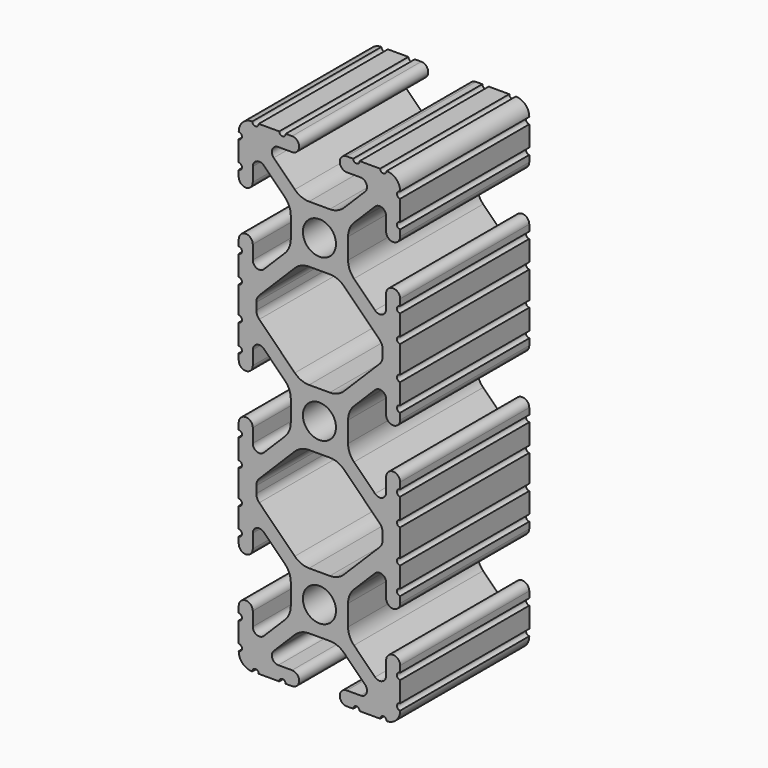
from build123d import *

# Parameters (mm, degrees)
F1_DEPTH = 25.4


# Not quite as in the source:
# - ends of sketch curves that miss each other by under 0.0002 mm in the source are joined


with BuildPart() as f1:
    # F0 (on Front) → F1 (new body)
    with BuildSketch(Plane.XZ):
        with BuildLine():
            ThreePointArc((-9.5504, 38.1), (-10.0584, 37.592), (-10.5664, 38.1))
            ThreePointArc((-10.5664, 38.1), (-12.0826749161, 37.4826749161), (-12.699997541, 35.9664000298))
            ThreePointArc((-12.699997541, 35.9664000298), (-12.192, 35.4584), (-12.7, 34.9504))
            Line((-12.7, 34.9504), (-12.7, 31.7246))
            ThreePointArc((-12.7, 31.7246), (-12.192, 31.2166), (-12.7, 30.7086))
            Line((-12.7, 30.7086), (-12.7, 29.7023028))
            ThreePointArc((-12.7, 29.7023028), (-11.5951, 28.5974028), (-10.4902, 29.7023028))
            Line((-10.4902, 29.7023028), (-10.4902, 31.8747902))
            ThreePointArc((-10.4902, 31.8747902), (-9.8630063673, 32.813451805), (-8.7557795103, 32.5932106897))
            Line((-8.7557795103, 32.5932106897), (-5.4384448, 29.2758622))
            ThreePointArc((-5.4384448, 29.2758622), (-4.7501824843, 28.2458268978), (-4.5085, 27.030807))
            Line((-4.5085, 27.030807), (-4.5085, 23.769193))
            ThreePointArc((-4.5085, 23.769193), (-4.7501824843, 22.5541731022), (-5.4384359697, 21.5241289697))
            Line((-5.4384359697, 21.5241289697), (-8.7557864, 18.2067962))
            ThreePointArc((-8.7557864, 18.2067962), (-9.8630063673, 17.986548195), (-10.4902, 18.9252098))
            Line((-10.4902, 18.9252098), (-10.4902, 21.0976972))
            ThreePointArc((-10.4902, 21.0976972), (-11.5951, 22.2025972), (-12.7, 21.0976972))
            Line((-12.7, 21.0976972), (-12.7, 20.0914))
            ThreePointArc((-12.7, 20.0914), (-12.192, 19.5834), (-12.7, 19.0754))
            Line((-12.7, 19.0754), (-12.7, 15.8496))
            ThreePointArc((-12.7, 15.8496), (-12.192, 15.3416), (-12.7, 14.8336))
            Line((-12.7, 14.8336), (-12.7, 10.5664))
            ThreePointArc((-12.7, 10.5664), (-12.192, 10.0584), (-12.7, 9.5504))
            Line((-12.7, 9.5504), (-12.7, 6.3246))
            ThreePointArc((-12.7, 6.3246), (-12.192, 5.8166), (-12.7, 5.3086))
            Line((-12.7, 5.3086), (-12.7, 4.3023028))
            ThreePointArc((-12.7, 4.3023028), (-11.5951, 3.1974028), (-10.4902, 4.3023028))
            Line((-10.4902, 4.3023028), (-10.4902, 6.4747902))
            ThreePointArc((-10.4902, 6.4747902), (-9.8630063673, 7.413451805), (-8.7557795103, 7.1932106897))
            Line((-8.7557795103, 7.1932106897), (-5.4384448, 3.8758622))
            ThreePointArc((-5.4384448, 3.8758622), (-4.7501824843, 2.8458268978), (-4.5085, 1.630807))
            Line((-4.5085, 1.630807), (-4.5085, -1.630807))
            ThreePointArc((-4.5085, -1.630807), (-4.7501824843, -2.8458268978), (-5.4384359697, -3.8758710303))
            Line((-5.4384359697, -3.8758710303), (-8.7557864, -7.1932038))
            ThreePointArc((-8.7557864, -7.1932038), (-9.8630063673, -7.413451805), (-10.4902, -6.4747902))
            Line((-10.4902, -6.4747902), (-10.4902, -4.3023028))
            ThreePointArc((-10.4902, -4.3023028), (-11.5951, -3.1974028), (-12.7, -4.3023028))
            Line((-12.7, -4.3023028), (-12.7, -5.3086))
            ThreePointArc((-12.7, -5.3086), (-12.192, -5.8166), (-12.7, -6.3246))
            Line((-12.7, -6.3246), (-12.7, -9.5504))
            ThreePointArc((-12.7, -9.5504), (-12.192, -10.0584), (-12.7, -10.5664))
            Line((-12.7, -10.5664), (-12.7, -14.8336))
            ThreePointArc((-12.7, -14.8336), (-12.192, -15.3416), (-12.7, -15.8496))
            Line((-12.7, -15.8496), (-12.7, -19.0754))
            ThreePointArc((-12.7, -19.0754), (-12.192, -19.5834), (-12.7, -20.0914))
            Line((-12.7, -20.0914), (-12.7, -21.0976972))
            ThreePointArc((-12.7, -21.0976972), (-11.5951, -22.2025972), (-10.4902, -21.0976972))
            Line((-10.4902, -21.0976972), (-10.4902, -18.9252098))
            ThreePointArc((-10.4902, -18.9252098), (-9.8630063673, -17.986548195), (-8.7557795103, -18.2067893103))
            Line((-8.7557795103, -18.2067893103), (-5.4384448, -21.5241378))
            ThreePointArc((-5.4384448, -21.5241378), (-4.7501824843, -22.5541731022), (-4.5085, -23.769193))
            Line((-4.5085, -23.769193), (-4.5085, -27.030807))
            ThreePointArc((-4.5085, -27.030807), (-4.7501824843, -28.2458268978), (-5.4384359697, -29.2758710303))
            Line((-5.4384359697, -29.2758710303), (-8.7557864, -32.5932038))
            ThreePointArc((-8.7557864, -32.5932038), (-9.8630063673, -32.813451805), (-10.4902, -31.8747902))
            Line((-10.4902, -31.8747902), (-10.4902, -29.7023028))
            ThreePointArc((-10.4902, -29.7023028), (-11.5951, -28.5974028), (-12.7, -29.7023028))
            Line((-12.7, -29.7023028), (-12.7, -30.7086))
            ThreePointArc((-12.7, -30.7086), (-12.192, -31.2166), (-12.7, -31.7246))
            Line((-12.7, -31.7246), (-12.7, -34.9504))
            ThreePointArc((-12.7, -34.9504), (-12.192, -35.4584), (-12.7, -35.9664))
            ThreePointArc((-12.7, -35.9664), (-12.0826749161, -37.4826749161), (-10.5664000298, -38.099997541))
            ThreePointArc((-10.5664000298, -38.099997541), (-10.0584, -37.592), (-9.5504, -38.1))
            Line((-9.5504, -38.1), (-6.3246, -38.1))
            ThreePointArc((-6.3246, -38.1), (-5.8166, -37.592), (-5.3086, -38.1))
            Line((-5.3086, -38.1), (-4.3023028, -38.1))
            ThreePointArc((-4.3023028, -38.1), (-3.1974028, -36.9951), (-4.3023028, -35.8902))
            Line((-4.3023028, -35.8902), (-6.4747902, -35.8902))
            ThreePointArc((-6.4747902, -35.8902), (-7.413451805, -35.2630063673), (-7.1932106897, -34.1557795103))
            Line((-7.1932106897, -34.1557795103), (-3.8758622, -30.8384448))
            ThreePointArc((-3.8758622, -30.8384448), (-2.8458268978, -30.1501824843), (-1.630807, -29.9085))
            Line((-1.630807, -29.9085), (1.630807, -29.9085))
            ThreePointArc((1.630807, -29.9085), (2.8458268978, -30.1501824843), (3.8758710303, -30.8384359697))
            Line((3.8758710303, -30.8384359697), (7.1932038, -34.1557864))
            ThreePointArc((7.1932038, -34.1557864), (7.413451805, -35.2630063673), (6.4747902, -35.8902))
            Line((6.4747902, -35.8902), (4.3023028, -35.8902))
            ThreePointArc((4.3023028, -35.8902), (3.1974028, -36.9951), (4.3023028, -38.1))
            Line((4.3023028, -38.1), (5.3086, -38.1))
            ThreePointArc((5.3086, -38.1), (5.8166, -37.592), (6.3246, -38.1))
            Line((6.3246, -38.1), (9.5504, -38.1))
            ThreePointArc((9.5504, -38.1), (10.0584, -37.592), (10.5664, -38.1))
            ThreePointArc((10.5664, -38.1), (12.0826749161, -37.4826749161), (12.699997541, -35.9664000298))
            ThreePointArc((12.699997541, -35.9664000298), (12.192, -35.4584), (12.7, -34.9504))
            Line((12.7, -34.9504), (12.7, -31.7246))
            ThreePointArc((12.7, -31.7246), (12.192, -31.2166), (12.7, -30.7086))
            Line((12.7, -30.7086), (12.7, -29.7023028))
            ThreePointArc((12.7, -29.7023028), (11.5951, -28.5974028), (10.4902, -29.7023028))
            Line((10.4902, -29.7023028), (10.4902, -31.8747902))
            ThreePointArc((10.4902, -31.8747902), (9.8630063673, -32.813451805), (8.7557795103, -32.5932106897))
            Line((8.7557795103, -32.5932106897), (5.4384448, -29.2758622))
            ThreePointArc((5.4384448, -29.2758622), (4.7501824843, -28.2458268978), (4.5085, -27.030807))
            Line((4.5085, -27.030807), (4.5085, -23.769193))
            ThreePointArc((4.5085, -23.769193), (4.7501824843, -22.5541731022), (5.4384359697, -21.5241289697))
            Line((5.4384359697, -21.5241289697), (8.7557864, -18.2067962))
            ThreePointArc((8.7557864, -18.2067962), (9.8630063673, -17.986548195), (10.4902, -18.9252098))
            Line((10.4902, -18.9252098), (10.4902, -21.0976972))
            ThreePointArc((10.4902, -21.0976972), (11.5951, -22.2025972), (12.7, -21.0976972))
            Line((12.7, -21.0976972), (12.7, -20.0914))
            ThreePointArc((12.7, -20.0914), (12.192, -19.5834), (12.7, -19.0754))
            Line((12.7, -19.0754), (12.7, -15.8496))
            ThreePointArc((12.7, -15.8496), (12.192, -15.3416), (12.7, -14.8336))
            Line((12.7, -14.8336), (12.7, -10.5664))
            ThreePointArc((12.7, -10.5664), (12.192, -10.0584), (12.7, -9.5504))
            Line((12.7, -9.5504), (12.7, -6.3246))
            ThreePointArc((12.7, -6.3246), (12.192, -5.8166), (12.7, -5.3086))
            Line((12.7, -5.3086), (12.7, -4.3023028))
            ThreePointArc((12.7, -4.3023028), (11.5951, -3.1974028), (10.4902, -4.3023028))
            Line((10.4902, -4.3023028), (10.4902, -6.4747902))
            ThreePointArc((10.4902, -6.4747902), (9.8630063673, -7.413451805), (8.7557795103, -7.1932106897))
            Line((8.7557795103, -7.1932106897), (5.4384448, -3.8758622))
            ThreePointArc((5.4384448, -3.8758622), (4.7501824843, -2.8458268978), (4.5085, -1.630807))
            Line((4.5085, -1.630807), (4.5085, 1.630807))
            ThreePointArc((4.5085, 1.630807), (4.7501824843, 2.8458268978), (5.4384359697, 3.8758710303))
            Line((5.4384359697, 3.8758710303), (8.7557864, 7.1932038))
            ThreePointArc((8.7557864, 7.1932038), (9.8630063673, 7.413451805), (10.4902, 6.4747902))
            Line((10.4902, 6.4747902), (10.4902, 4.3023028))
            ThreePointArc((10.4902, 4.3023028), (11.5951, 3.1974028), (12.7, 4.3023028))
            Line((12.7, 4.3023028), (12.7, 5.3086))
            ThreePointArc((12.7, 5.3086), (12.192, 5.8166), (12.7, 6.3246))
            Line((12.7, 6.3246), (12.7, 9.5504))
            ThreePointArc((12.7, 9.5504), (12.192, 10.0584), (12.7, 10.5664))
            Line((12.7, 10.5664), (12.7, 14.8336))
            ThreePointArc((12.7, 14.8336), (12.192, 15.3416), (12.7, 15.8496))
            Line((12.7, 15.8496), (12.7, 19.0754))
            ThreePointArc((12.7, 19.0754), (12.192, 19.5834), (12.7, 20.0914))
            Line((12.7, 20.0914), (12.7, 21.0976972))
            ThreePointArc((12.7, 21.0976972), (11.5951, 22.2025972), (10.4902, 21.0976972))
            Line((10.4902, 21.0976972), (10.4902, 18.9252098))
            ThreePointArc((10.4902, 18.9252098), (9.8630063673, 17.986548195), (8.7557795103, 18.2067893103))
            Line((8.7557795103, 18.2067893103), (5.4384448, 21.5241378))
            ThreePointArc((5.4384448, 21.5241378), (4.7501824843, 22.5541731022), (4.5085, 23.769193))
            Line((4.5085, 23.769193), (4.5085, 27.030807))
            ThreePointArc((4.5085, 27.030807), (4.7501824843, 28.2458268978), (5.4384359697, 29.2758710303))
            Line((5.4384359697, 29.2758710303), (8.7557864, 32.5932038))
            ThreePointArc((8.7557864, 32.5932038), (9.8630063673, 32.813451805), (10.4902, 31.8747902))
            Line((10.4902, 31.8747902), (10.4902, 29.7023028))
            ThreePointArc((10.4902, 29.7023028), (11.5951, 28.5974028), (12.7, 29.7023028))
            Line((12.7, 29.7023028), (12.7, 30.7086))
            ThreePointArc((12.7, 30.7086), (12.192, 31.2166), (12.7, 31.7246))
            Line((12.7, 31.7246), (12.7, 34.9504))
            ThreePointArc((12.7, 34.9504), (12.192, 35.4584), (12.7, 35.9664))
            ThreePointArc((12.7, 35.9664), (12.0826749161, 37.4826749161), (10.5664000298, 38.099997541))
            ThreePointArc((10.5664000298, 38.099997541), (10.0584, 37.592), (9.5504, 38.1))
            Line((9.5504, 38.1), (6.3246, 38.1))
            ThreePointArc((6.3246, 38.1), (5.8166, 37.592), (5.3086, 38.1))
            Line((5.3086, 38.1), (4.3023028, 38.1))
            ThreePointArc((4.3023028, 38.1), (3.1974028, 36.9951), (4.3023028, 35.8902))
            Line((4.3023028, 35.8902), (6.4747902, 35.8902))
            ThreePointArc((6.4747902, 35.8902), (7.413451805, 35.2630063673), (7.1932106897, 34.1557795103))
            Line((7.1932106897, 34.1557795103), (3.8758622, 30.8384448))
            ThreePointArc((3.8758622, 30.8384448), (2.8458268978, 30.1501824843), (1.630807, 29.9085))
            Line((1.630807, 29.9085), (-1.630807, 29.9085))
            ThreePointArc((-1.630807, 29.9085), (-2.8458268978, 30.1501824843), (-3.8758710303, 30.8384359697))
            Line((-3.8758710303, 30.8384359697), (-7.1932038, 34.1557864))
            ThreePointArc((-7.1932038, 34.1557864), (-7.413451805, 35.2630063673), (-6.4747902, 35.8902))
            Line((-6.4747902, 35.8902), (-4.3023028, 35.8902))
            ThreePointArc((-4.3023028, 35.8902), (-3.1974028, 36.9951), (-4.3023028, 38.1))
            Line((-4.3023028, 38.1), (-5.3086, 38.1))
            ThreePointArc((-5.3086, 38.1), (-5.8166, 37.592), (-6.3246, 38.1))
            Line((-6.3246, 38.1), (-9.5504, 38.1))
        make_face()
        with BuildLine():
            ThreePointArc((-2.6035, -25.4), (0, -22.7965), (2.6035, -25.4))
            ThreePointArc((2.6035, -25.4), (0, -28.0035), (-2.6035, -25.4))
        make_face(mode=Mode.SUBTRACT)
        with BuildLine():
            Line((-9.4701614, -11.0327186), (-3.8758622, -5.4384448))
            ThreePointArc((-3.8758622, -5.4384448), (-2.8458268978, -4.7501824843), (-1.630807, -4.5085))
            Line((-1.630807, -4.5085), (1.630807, -4.5085))
            ThreePointArc((1.630807, -4.5085), (2.8458268978, -4.7501824843), (3.8758710303, -5.4384359697))
            Line((3.8758710303, -5.4384359697), (9.4701614, -11.0327186))
            ThreePointArc((9.4701614, -11.0327186), (9.8115254878, -11.5436301307), (9.9314, -12.14628))
            Line((9.9314, -12.14628), (9.9314, -13.25372))
            ThreePointArc((9.9314, -13.25372), (9.8115254878, -13.8563698693), (9.470151759, -14.367271759))
            Line((9.470151759, -14.367271759), (3.8758622, -19.9615552))
            ThreePointArc((3.8758622, -19.9615552), (2.8458268978, -20.6498175157), (1.630807, -20.8915))
            Line((1.630807, -20.8915), (-1.630807, -20.8915))
            ThreePointArc((-1.630807, -20.8915), (-2.8458268978, -20.6498175157), (-3.8758710303, -19.9615640303))
            Line((-3.8758710303, -19.9615640303), (-9.4701614, -14.3672814))
            ThreePointArc((-9.4701614, -14.3672814), (-9.8115254878, -13.8563698693), (-9.9314, -13.25372))
            Line((-9.9314, -13.25372), (-9.9314, -12.14628))
            ThreePointArc((-9.9314, -12.14628), (-9.8115254878, -11.5436301307), (-9.4701614, -11.0327186))
        make_face(mode=Mode.SUBTRACT)
        with BuildLine():
            ThreePointArc((-2.6035, 0), (0, 2.6035), (2.6035, 0))
            ThreePointArc((2.6035, 0), (0, -2.6035), (-2.6035, 0))
        make_face(mode=Mode.SUBTRACT)
        with BuildLine():
            Line((-9.4701614, 14.3672814), (-3.8758622, 19.9615552))
            ThreePointArc((-3.8758622, 19.9615552), (-2.8458268978, 20.6498175157), (-1.630807, 20.8915))
            Line((-1.630807, 20.8915), (1.630807, 20.8915))
            ThreePointArc((1.630807, 20.8915), (2.8458268978, 20.6498175157), (3.8758710303, 19.9615640303))
            Line((3.8758710303, 19.9615640303), (9.4701614, 14.3672814))
            ThreePointArc((9.4701614, 14.3672814), (9.8115254878, 13.8563698693), (9.9314, 13.25372))
            Line((9.9314, 13.25372), (9.9314, 12.14628))
            ThreePointArc((9.9314, 12.14628), (9.8115254878, 11.5436301307), (9.470151759, 11.032728241))
            Line((9.470151759, 11.032728241), (3.8758622, 5.4384448))
            ThreePointArc((3.8758622, 5.4384448), (2.8458268978, 4.7501824843), (1.630807, 4.5085))
            Line((1.630807, 4.5085), (-1.630807, 4.5085))
            ThreePointArc((-1.630807, 4.5085), (-2.8458268978, 4.7501824843), (-3.8758710303, 5.4384359697))
            Line((-3.8758710303, 5.4384359697), (-9.4701614, 11.0327186))
            ThreePointArc((-9.4701614, 11.0327186), (-9.8115254878, 11.5436301307), (-9.9314, 12.14628))
            Line((-9.9314, 12.14628), (-9.9314, 13.25372))
            ThreePointArc((-9.9314, 13.25372), (-9.8115254878, 13.8563698693), (-9.4701614, 14.3672814))
        make_face(mode=Mode.SUBTRACT)
        with BuildLine():
            ThreePointArc((-2.6035, 25.4), (0, 28.0035), (2.6035, 25.4))
            ThreePointArc((2.6035, 25.4), (0, 22.7965), (-2.6035, 25.4))
        make_face(mode=Mode.SUBTRACT)
    extrude(amount=F1_DEPTH)


solid = f1.part
